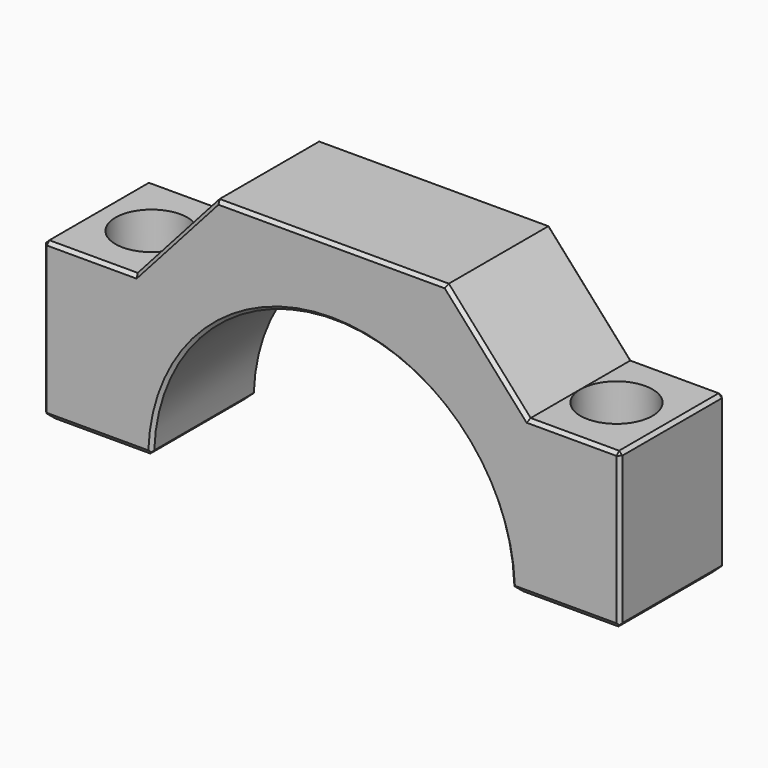
from build123d import *

# Parameters (mm, degrees)
F1_DEPTH    = 20
F3_D        = 6.6
F5_D        = 11
F5_DEPTH    = 6.4
F5_TIP      = 3.3047334047
F7_D        = 11
F7_DEPTH    = 6.4
F7_TIP      = 3.3047334047
F8_T1_DEPTH = 21.6433659759
F8_T3_DEPTH = 25.1433659759
F8_T5_DEPTH = 21.6433659759
F8_T7_DEPTH = 25.0580427678
F9_SIZE     = 0.5


# Not quite as in the source:
# - a fillet or chamfer that OpenCascade refuses, or shapes differently, is made with other operations: its cross-section is extruded or revolved along the edge and cut away or added


with BuildPart() as f1:
    # F0 (on Front) → F1 (new body)
    with BuildSketch(Plane.XZ):
        with BuildLine():
            ThreePointArc((-27.5, 0), (0, 27.5), (27.5, 0))
            Line((27.5, 0), (44, 0))
            Line((44, 0), (44, 24))
            Line((44, 24), (30, 24))
            Line((30, 24), (17.5, 38))
            Line((17.5, 38), (-17.5, 38))
            Line((-17.5, 38), (-30, 24))
            Line((-30, 24), (-44, 24))
            Line((-44, 24), (-44, 0))
            Line((-44, 0), (-27.5, 0))
        make_face()
    extrude(amount=F1_DEPTH)

    # F3 (through all)
    with Locations(Plane(origin=(0, 0, 0), x_dir=(1, 0, 0), z_dir=(0, 0, -1))):
        with Locations((-35.5, 10), (35.5, 10)):
            Hole(F3_D / 2)

    # F5
    with Locations(Plane.XY.offset(24)):
        with Locations((-35.5, -10)):
            Hole(F5_D / 2, depth=F5_DEPTH)
            with Locations((0, 0, -(F5_DEPTH + F5_TIP / 2))):  # 118° drill point
                Cone(0, F5_D / 2, F5_TIP, mode=Mode.SUBTRACT)

    # F7
    with Locations(Plane.XY.offset(24)):
        with Locations((35.5, -10)):
            Hole(F7_D / 2, depth=F7_DEPTH)
            with Locations((0, 0, -(F7_DEPTH + F7_TIP / 2))):  # 118° drill point
                Cone(0, F7_D / 2, F7_TIP, mode=Mode.SUBTRACT)

    # F8: chamfer of 1 on 8 edges, made by hand

    # F8_s2 → F8_t1 (cut)
    with BuildSketch(Plane.YZ.offset(24.928317012)):
        Polygon((-19, 0), (-20, 1), (-20, 0), align=None)
        Polygon((-1, 0), (0, 1), (0, 0), align=None)
    extrude(amount=F8_T1_DEPTH, mode=Mode.SUBTRACT)

    # F8_s4 → F8_t3 (cut)
    with BuildSketch(Plane.XZ.offset(-2.571682988)):
        Polygon((43, 0), (44, 1), (44, 0), align=None)
        Polygon((-43, 0), (-44, 1), (-44, 0), align=None)
    extrude(amount=F8_T3_DEPTH, mode=Mode.SUBTRACT)

    # F8_s6 → F8_t5 (cut)
    with BuildSketch(Plane.YZ.offset(-46.571682988)):
        Polygon((-19, 0), (-20, 1), (-20, 0), align=None)
        Polygon((-1, 0), (0, 1), (0, 0), align=None)
    extrude(amount=F8_T5_DEPTH, mode=Mode.SUBTRACT)

    # F8_s8 → F8_t7 (cut)
    with BuildSketch(Plane.XZ.offset(-2.5290213839)):
        with BuildLine():
            Line((-27.4830665009, 0.9649122807), (-28.4824507373, 0))
            Line((-28.4824507373, 0), (-27.5, 0))
            ThreePointArc((-27.5, 0), (-27.4955143469, 0.4966797747), (-27.4830665009, 0.9649122807))
        make_face()
        with BuildLine():
            Line((27.4830665009, 0.9649122807), (28.4824507373, 0))
            Line((28.4824507373, 0), (27.5, 0))
            ThreePointArc((27.5, 0), (27.4955143469, 0.4966797747), (27.4830665009, 0.9649122807))
        make_face()
    extrude(amount=F8_T7_DEPTH, mode=Mode.SUBTRACT)

    # F9
    f9_edges = [f1.edges().sort_by_distance(p)[0] for p in [
        (44, -20, 12.5),
        (44, 0, 12.5),
        (44, -10, 24),
        (37, -20, 24),
        (37, 0, 24),
        (23.75, 0, 31),
        (23.75, -20, 31),
        (0, -20, 38),
        (0, 0, 38),
        (-23.75, -20, 31),
        (0, -20, 27.5),
        (-44, -20, 12.5),
        (-37, -20, 24),
        (-44, -10, 24),
        (-37, 0, 24),
        (0, 0, 27.5),
        (-23.75, 0, 31),
        (-44, 0, 12.5),
    ]]
    chamfer(f9_edges, length=F9_SIZE)


solid = f1.part
